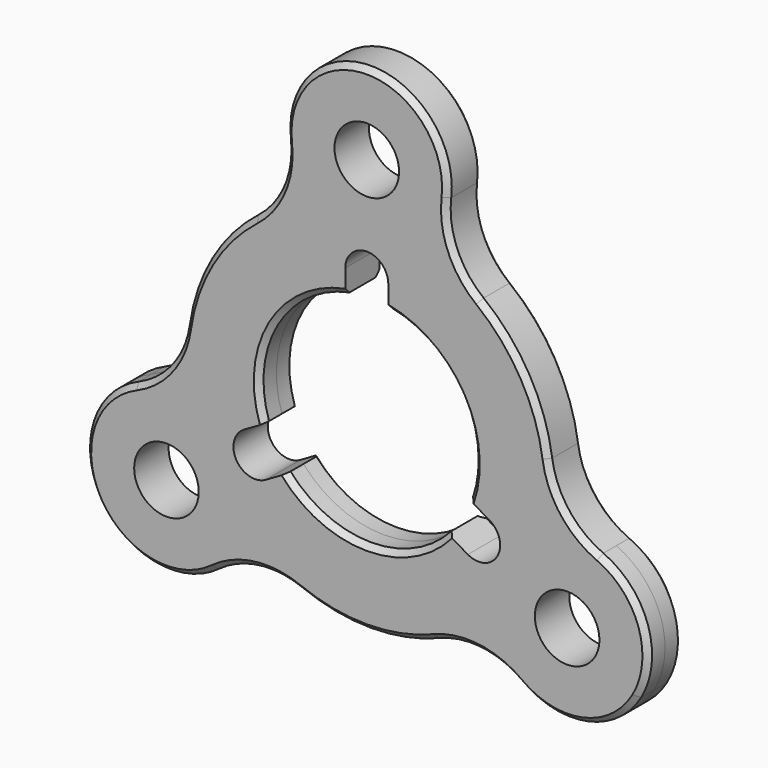
from build123d import *

# Parameters (mm, degrees)
F0_R          = 10
F1_DEPTH      = 2
F1_DEPTH_BACK = 2
F3_D          = 6
F4_SIZE       = 0.5
F7_DEPTH      = 4.001


# Not quite as in the source:
# - two fillets or chamfers of one size are made in one step


with BuildPart() as f1:
    # F0 (on Front) → F1 (new body, two sides)
    with BuildSketch(Plane.XZ) as f1_sk:
        with BuildLine():
            ThreePointArc((10.4685027699, 13.3944186047), (8.0122088596, 16.6160342353), (7.4491243619, 20.6279069767))
            ThreePointArc((7.4491243619, 20.6279069767), (5.6031552573, 26.4854439284), (0, 29))
            ThreePointArc((0, 29), (-5.6031552573, 26.4854439284), (-7.4491243619, 20.6279069767))
            ThreePointArc((-7.4491243619, 20.6279069767), (-8.0122088596, 16.6160342353), (-10.4685027699, 13.3944186047))
            ThreePointArc((-10.4685027699, 13.3944186047), (-14.7224318643, 8.5), (-16.8341581655, 2.368780036))
            ThreePointArc((-16.8341581655, 2.368780036), (-18.3960121877, -1.3692407048), (-21.5888536497, -3.862822555))
            ThreePointArc((-21.5888536497, -3.862822555), (-25.7386449011, -8.39024717), (-25.1147367097, -14.5))
            ThreePointArc((-25.1147367097, -14.5), (-20.1354896438, -18.0951967583), (-14.1397292878, -16.7650844217))
            ThreePointArc((-14.1397292878, -16.7650844217), (-10.3838033281, -15.2467935304), (-6.3656553956, -15.7631986406))
            ThreePointArc((-6.3656553956, -15.7631986406), (0, -17), (6.3656553956, -15.7631986406))
            ThreePointArc((6.3656553956, -15.7631986406), (10.3838033281, -15.2467935304), (14.1397292878, -16.7650844217))
            ThreePointArc((14.1397292878, -16.7650844217), (20.1354896438, -18.0951967583), (25.1147367097, -14.5))
            ThreePointArc((25.1147367097, -14.5), (25.7386449011, -8.39024717), (21.5888536497, -3.862822555))
            ThreePointArc((21.5888536497, -3.862822555), (18.3960121877, -1.3692407048), (16.8341581655, 2.368780036))
            ThreePointArc((16.8341581655, 2.368780036), (14.7224318643, 8.5), (10.4685027699, 13.3944186047))
        make_face()
        Circle(F0_R, mode=Mode.SUBTRACT)
    extrude(amount=F1_DEPTH)
    extrude(f1_sk.sketch, amount=-F1_DEPTH_BACK)

    # F3 (through all)
    with Locations(Plane.XZ.offset(2)):
        with Locations((0, 21.5), (-18.6195461814, -10.75), (18.6195461814, -10.75)):
            Hole(F3_D / 2)

    # F4
    f4_edges = [f1.edges().sort_by_distance(p)[0] for p in [
        (-10, -2, 0),
        (10, 0, 0),
        (-10, 2, 0),
        (8.012209, -2, 16.616034),
        (8.012209, 2, 16.616034),
        (14.722432, -2, 8.5),
        (14.722432, 2, 8.5),
        (0, -2, 29),
        (18.396012, -2, -1.369241),
        (-8.012209, -2, 16.616034),
        (25.114737, -2, -14.5),
        (-14.722432, -2, 8.5),
        (10.383803, -2, -15.246794),
        (-18.396012, -2, -1.369241),
        (0, -2, -17),
        (-25.114737, -2, -14.5),
        (-10.383803, -2, -15.246794),
        (0, 2, 29),
        (18.396012, 2, -1.369241),
        (-8.012209, 2, 16.616034),
        (25.114737, 2, -14.5),
        (-14.722432, 2, 8.5),
        (10.383803, 2, -15.246794),
        (-18.396012, 2, -1.369241),
        (0, 2, -17),
        (-25.114737, 2, -14.5),
        (-10.383803, 2, -15.246794),
    ]]
    chamfer(f4_edges, length=F4_SIZE)

    # F6 (on face) → F7 (cut, through all)
    with BuildSketch(Plane(origin=(0, 2, 0), x_dir=(-1, 0, 0), z_dir=(0, 1, 0))):
        with BuildLine():
            ThreePointArc((-2, 9.7979589711), (0, 10), (2, 9.7979589711))
            Line((2, 9.7979589711), (2, 12))
            ThreePointArc((2, 12), (0, 14), (-2, 12))
            Line((-2, 12), (-2, 9.7979589711))
        make_face()
        with BuildLine():
            Line((-9.3923048454, -7.7320508076), (-7.4852813742, -6.6310302931))
            ThreePointArc((-7.4852813742, -6.6310302931), (-8.6602540378, -5), (-9.4852813742, -3.166928678))
            Line((-9.4852813742, -3.166928678), (-11.3923048454, -4.2679491924))
            ThreePointArc((-11.3923048454, -4.2679491924), (-12.124355653, -7), (-9.3923048454, -7.7320508076))
        make_face()
        with BuildLine():
            Line((11.3923048454, -4.2679491924), (9.4852813742, -3.166928678))
            ThreePointArc((9.4852813742, -3.166928678), (8.6602540378, -5), (7.4852813742, -6.6310302931))
            Line((7.4852813742, -6.6310302931), (9.3923048454, -7.7320508076))
            ThreePointArc((9.3923048454, -7.7320508076), (12.124355653, -7), (11.3923048454, -4.2679491924))
        make_face()
    extrude(amount=-F7_DEPTH, mode=Mode.SUBTRACT)


solid = f1.part
